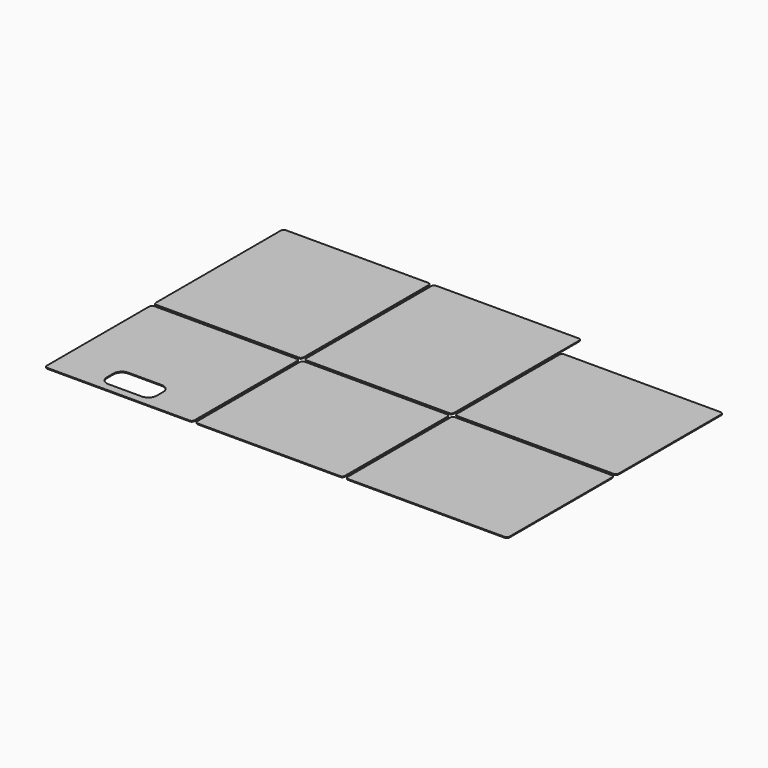
from build123d import *

# Parameters (mm, degrees)
F1_DEPTH = 3.175


# Not quite as in the source:
# - a length typed as a fraction of an inch, garbled in the dataset ("3 / 203.2 mm" for 3/8 in), is restored
# - a feature names something its author has since deleted; it is built from what else it names


with BuildPart() as f1:
    # F0 (on Top) → F1 (new body)
    with BuildSketch(Plane.XY):
        with BuildLine():
            Line((-10, 1076.8), (-523.4, 1076.8))
            ThreePointArc((-523.4, 1076.8), (-530.4710678119, 1073.8710678119), (-533.4, 1066.8))
            Line((-533.4, 1066.8), (-533.4, 502.6))
            ThreePointArc((-533.4, 502.6), (-530.4710678119, 495.5289321881), (-523.4, 492.6))
            Line((-523.4, 492.6), (-10, 492.6))
            ThreePointArc((-10, 492.6), (-2.9289321881, 495.5289321881), (0, 502.6))
            Line((0, 502.6), (0, 1066.8))
            ThreePointArc((0, 1066.8), (-2.9289321881, 1073.8710678119), (-10, 1076.8))
        make_face()
    extrude(amount=F1_DEPTH)


with BuildPart() as f1b:
    # F0 (on Top) → F1, piece 2 (new body)
    with BuildSketch(Plane.XY):
        with BuildLine():
            Line((-10, 482.6), (-523.4, 482.6))
            ThreePointArc((-523.4, 482.6), (-530.4710678119, 479.6710678119), (-533.4, 472.6))
            Line((-533.4, 472.6), (-533.4, 10))
            ThreePointArc((-533.4, 10), (-530.4710678119, 2.9289321881), (-523.4, 0))
            Line((-523.4, 0), (-10, 0))
            ThreePointArc((-10, 0), (-2.9289321881, 2.9289321881), (0, 10))
            Line((0, 10), (0, 472.6))
            ThreePointArc((0, 472.6), (-2.9289321881, 479.6710678119), (-10, 482.6))
        make_face()
    extrude(amount=F1_DEPTH)


with BuildPart() as f1c:
    # F0 (on Top) → F1, piece 3 (new body)
    with BuildSketch(Plane.XY):
        with BuildLine():
            Line((584.2, 482.6), (20, 482.6))
            ThreePointArc((20, 482.6), (12.9289321881, 479.6710678119), (10, 472.6))
            Line((10, 472.6), (10, 10))
            ThreePointArc((10, 10), (12.9289321881, 2.9289321881), (20, 0))
            Line((20, 0), (584.2, 0))
            ThreePointArc((584.2, 0), (591.2710678119, 2.9289321881), (594.2, 10))
            Line((594.2, 10), (594.2, 472.6))
            ThreePointArc((594.2, 472.6), (591.2710678119, 479.6710678119), (584.2, 482.6))
        make_face()
    extrude(amount=F1_DEPTH)


with BuildPart() as f1d:
    # F0 (on Top) → F1, piece 4 (new body)
    with BuildSketch(Plane.XY):
        with BuildLine():
            ThreePointArc((-543.4, 1066.8), (-546.3289321881, 1073.8710678119), (-553.4, 1076.8))
            Line((-553.4, 1076.8), (-1066.8, 1076.8))
            ThreePointArc((-1066.8, 1076.8), (-1073.8710678119, 1073.8710678119), (-1076.8, 1066.8))
            Line((-1076.8, 1066.8), (-1076.8, 502.6))
            ThreePointArc((-1076.8, 502.6), (-1073.8710678119, 495.5289321881), (-1066.8, 492.6))
            Line((-1066.8, 492.6), (-553.4, 492.6))
            ThreePointArc((-553.4, 492.6), (-546.3289321881, 495.5289321881), (-543.4, 502.6))
            Line((-543.4, 502.6), (-543.4, 1066.8))
        make_face()
    extrude(amount=F1_DEPTH)


with BuildPart() as f1e:
    # F0 (on Top) → F1, piece 5 (new body)
    with BuildSketch(Plane.XY):
        with BuildLine():
            Line((-1066.8, 0), (-553.4, 0))
            ThreePointArc((-553.4, 0), (-546.3289321881, 2.9289321881), (-543.4, 10))
            Line((-543.4, 10), (-543.4, 472.6))
            ThreePointArc((-543.4, 472.6), (-546.3289321881, 479.6710678119), (-553.4, 482.6))
            Line((-553.4, 482.6), (-1066.8, 482.6))
            ThreePointArc((-1066.8, 482.6), (-1073.8710678119, 479.6710678119), (-1076.8, 472.6))
            Line((-1076.8, 472.6), (-1076.8, 10))
            ThreePointArc((-1076.8, 10), (-1073.8710678119, 2.9289321881), (-1066.8, 0))
        make_face()
        with BuildLine():
            ThreePointArc((-900.1, 90), (-891.3132034356, 111.2132034356), (-870.1, 120))
            Line((-870.1, 120), (-750.1, 120))
            ThreePointArc((-750.1, 120), (-728.8867965644, 111.2132034356), (-720.1, 90))
            Line((-720.1, 90), (-720.1, 60))
            ThreePointArc((-720.1, 60), (-728.8867965644, 38.7867965644), (-750.1, 30))
            Line((-750.1, 30), (-870.1, 30))
            ThreePointArc((-870.1, 30), (-891.3132034356, 38.7867965644), (-900.1, 60))
            Line((-900.1, 60), (-900.1, 90))
        make_face(mode=Mode.SUBTRACT)
    extrude(amount=F1_DEPTH)


with BuildPart() as f1f:
    # F0 (on Top) → F1, piece 6 (new body)
    with BuildSketch(Plane.XY):
        with BuildLine():
            ThreePointArc((10, 502.6), (12.9289321881, 495.5289321881), (20, 492.6))
            Line((20, 492.6), (584.2, 492.6))
            ThreePointArc((584.2, 492.6), (591.2710678119, 495.5289321881), (594.2, 502.6))
            Line((594.2, 502.6), (594.2, 965.2))
            ThreePointArc((594.2, 965.2), (591.2710678119, 972.2710678119), (584.2, 975.2))
            Line((584.2, 975.2), (20, 975.2))
            ThreePointArc((20, 975.2), (12.9289321881, 972.2710678119), (10, 965.2))
            Line((10, 965.2), (10, 502.6))
        make_face()
    extrude(amount=F1_DEPTH)


solid = Compound([f1.part, f1b.part, f1c.part, f1d.part, f1e.part, f1f.part])
